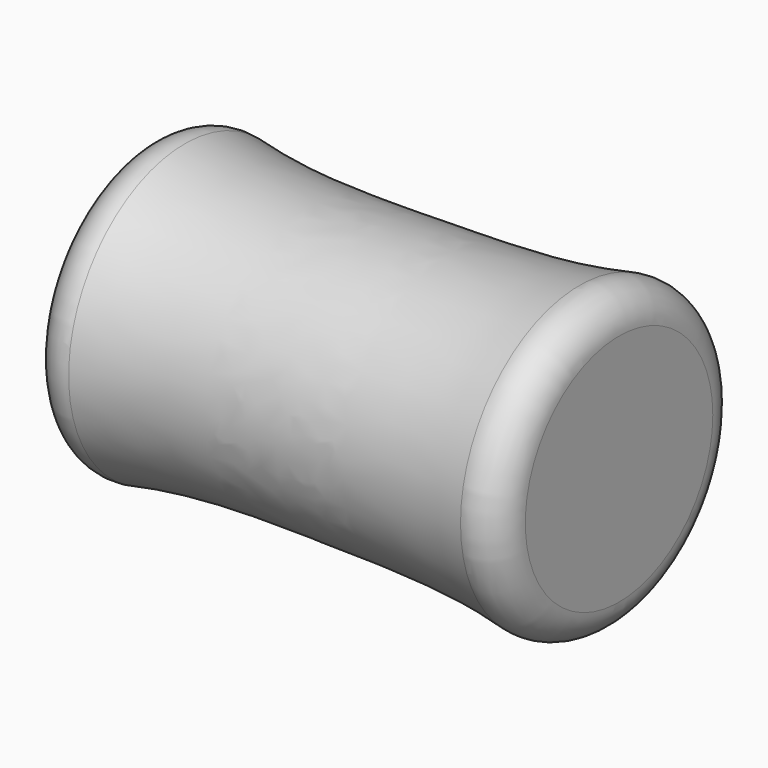
from build123d import *


with BuildPart() as f1:
    # F0 (on Top) → F1 (revolve)
    with BuildSketch(Plane.XY):
        with BuildLine():
            add(Edge.make_bspline(
                [(-39.5460653094, 36.326142192), (-26.6360909109, 33.6743616146), (0.573592198, 34.3413720973), (24.5421229151, 34.3794363135), (37.3864209129, 37.0661812385)],
                knots=[0.084198921, 0.084198921, 0.084198921, 0.084198921, 0.5055680854, 0.9192112313, 0.9192112313, 0.9192112313, 0.9192112313], degree=3))
            ThreePointArc((-39.5460653094, 36.326142192), (-44.8367833652, 35.0271623847), (-47.1737161279, 30.1060048635))
            Line((-47.1737161279, 30.1060048635), (-47.1737161279, 8.0222934484))
            Line((-47.1737161279, 8.0222934484), (45.0365617871, 8.0222934484))
            Line((45.0365617871, 8.0222934484), (45.0365617871, 30.8507058981))
            ThreePointArc((45.0365617871, 30.8507058981), (42.6907224638, 35.7791130724), (37.3864209129, 37.0661812385))
        make_face()
    revolve(axis=Axis((-1.0685771704, 8.0222934484, 0), (1, 0, 0)))


solid = f1.part
